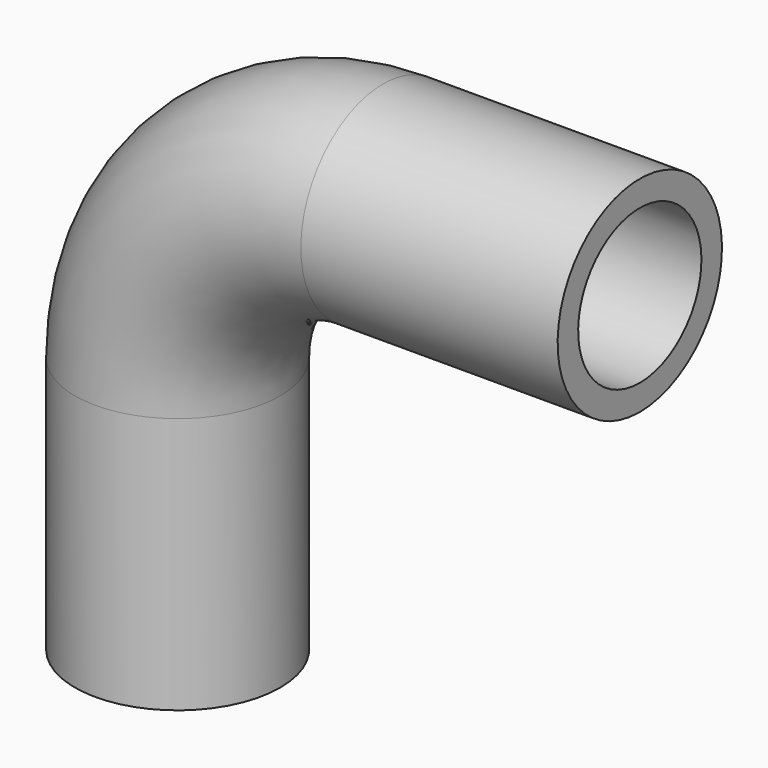
from build123d import *

# Parameters (mm, degrees)
F0_R     = 10
F0_R_2   = 7.5
F1_DEPTH = 25
F3_R     = 10
F3_R_2   = 7.5
F4_ANGLE = 90
F5_DEPTH = 25


with BuildPart() as f1:
    # F0 (on Top) → F1 (new body)
    with BuildSketch(Plane.XY):
        Circle(F0_R)
        Circle(F0_R_2, mode=Mode.SUBTRACT)
    extrude(amount=F1_DEPTH)

    # F3 (on face) → F4 (revolve)
    with BuildSketch(Plane.XY.offset(25)):
        Circle(F3_R)
        Circle(F3_R_2, mode=Mode.SUBTRACT)
    revolve(axis=Axis((20, 0.0099948445, 25), (0, 1, 0)), revolution_arc=F4_ANGLE)

    # F5 (add): a face of the model
    f5_faces = [f1.faces().sort_by_distance(p)[0] for p in [
        (20, 0, 54.7171572875),
    ]]
    extrude(f5_faces, amount=F5_DEPTH)


solid = f1.part
